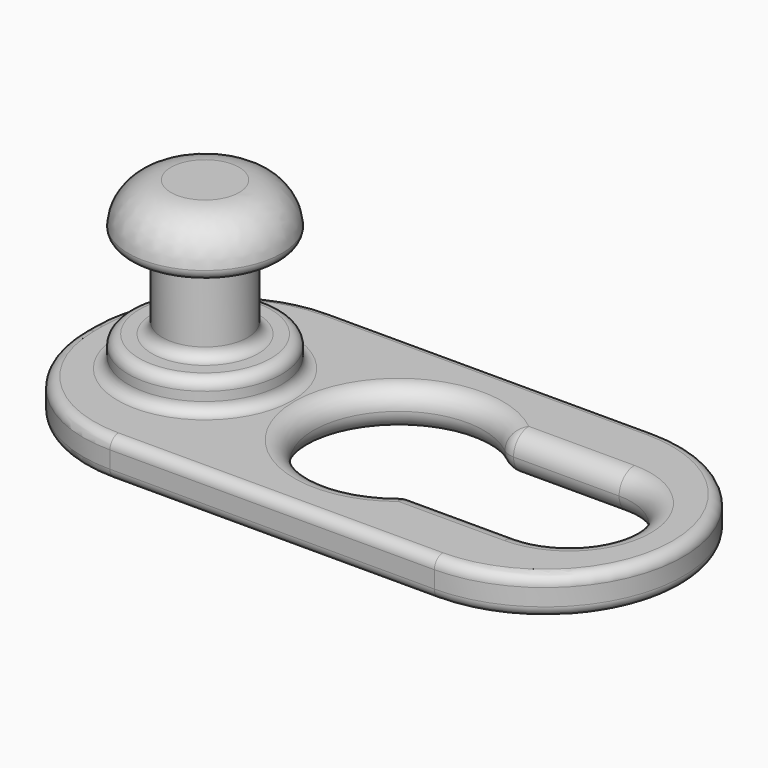
from build123d import *

# Parameters (mm, degrees)
F0_R     = 7.2
F1_DEPTH = 3.6
F2_R     = 1.79999
F3_R     = 7.2
F4_DEPTH = 6.45
F5_R     = 4
F6_DEPTH = 8
F8_R     = 1
F7_R     = 7.2
F7_R_2   = 4
F9_DEPTH = 4.75
F10_R    = 1
F12_R    = 1


# Not quite as in the source:
# - a fillet or chamfer that OpenCascade refuses, or shapes differently, is made with other operations: its cross-section is extruded or revolved along the edge and cut away or added
# - a fillet or chamfer is up to 0.001 mm smaller than in the source, because OpenCascade refuses the exact size


with BuildPart() as f1:
    # F0 (on Top) → F1 (new body)
    with BuildSketch(Plane.XY):
        with BuildLine():
            ThreePointArc((-17.2561568693, 13.0195750748), (-26.0949916342, 9.3584098397), (-29.7561568693, 0.5195750748))
            Line((-29.7561568693, 0.5195750748), (-29.7561568693, 0))
            Line((-29.7561568693, 0), (-29.7561568693, -0.4804249252))
            ThreePointArc((-29.7561568693, -0.4804249252), (-26.0949916342, -9.31925969), (-17.2561568693, -12.9804249252))
            Line((-17.2561568693, -12.9804249252), (13.2438431307, -12.9804249252))
            ThreePointArc((13.2438431307, -12.9804249252), (22.4362312861, -9.1728130806), (26.2438431307, 0.0195750748))
            ThreePointArc((26.2438431307, 0.0195750748), (22.4362312861, 9.2119632303), (13.2438431307, 13.0195750748))
            Line((13.2438431307, 13.0195750748), (-17.2561568693, 13.0195750748))
        make_face()
        with Locations((-18.7568739057, 0)):
            Circle(F0_R, mode=Mode.SUBTRACT)
        with BuildLine():
            ThreePointArc((4.956876454, -5.85), (-8.4999999419, 0), (4.956876454, 5.85))
            Line((4.956876454, 5.85), (5.4, 5.85))
            Line((5.4, 5.85), (15.5500000581, 5.85))
            ThreePointArc((15.5500000581, 5.85), (21.4000000581, 0), (15.5500000581, -5.85))
            Line((15.5500000581, -5.85), (5.4, -5.85))
            Line((5.4, -5.85), (4.956876454, -5.85))
        make_face(mode=Mode.SUBTRACT)
        with Locations((-18.7568739057, 0)):
            Circle(F0_R)
    extrude(amount=F1_DEPTH)

    # F2 (radius 1.8 in the source; OpenCascade refuses exactly that, so slightly less here)
    f2_edges = [f1.edges().sort_by_distance(p)[0] for p in [
        (4.956876, -5.85, 1.8),
        (4.956876, 5.85, 1.8),
        (-8.5, 0, 0),
        (-8.5, 0, 3.6),
        (15.55, 5.85, 1.8),
        (10.253438, 5.85, 0),
        (10.253438, 5.85, 3.6),
        (15.55, -5.85, 1.8),
        (21.4, 0, 0),
        (21.4, 0, 3.6),
        (10.253438, -5.85, 0),
        (10.253438, -5.85, 3.6),
    ]]
    fillet(f2_edges, radius=F2_R)

    # F3 (on Top) → F4 (join)
    with BuildSketch(Plane.XY):
        with Locations((-18.7010411173, 0)):
            Circle(F3_R)
    extrude(amount=F4_DEPTH)

    # F5 (on face) → F6 (join)
    with BuildSketch(Plane.XY.offset(6.45)):
        with Locations((-18.7010411173, 0)):
            Circle(F5_R)
    extrude(amount=F6_DEPTH)

    # F8
    f8_edges = [f1.edges().sort_by_distance(p)[0] for p in [
        (-25.901041, 0, 6.45),
        (-22.701041, 0, 6.45),
        (-25.901041, 0, 3.6),
        (-11.501041, 0, 5.025),
    ]]
    fillet(f8_edges, radius=F8_R)

    # F7 (on face) → F9 (join)
    with BuildSketch(Plane.XY.offset(14.45)):
        with Locations((-18.7010411173, 0)):
            Circle(F7_R)
        with Locations((-18.7010411173, 0)):
            Circle(F7_R_2, mode=Mode.SUBTRACT)
        with Locations((-18.7010411173, 0)):
            Circle(F7_R_2)
    extrude(amount=F9_DEPTH)

    # F10
    f10_edges = [f1.edges().sort_by_distance(p)[0] for p in [
        (-25.901041, 0, 14.45),
        (-22.701041, 0, 14.45),
        (-14.701041, 0, 10.95),
        (-22.701041, 0, 7.45),
    ]]
    fillet(f10_edges, radius=F10_R)

    # F11: fillet of radius 4 on 3 edges, made by hand

    # F11_s1 → F11_t2 (revolve, cut)
    with BuildSketch(Plane.XZ):
        with BuildLine():
            ThreePointArc((-11.5010411173, 15.45), (-12.7546081855, 18.1154759474), (-15.493220973, 19.2))
            Line((-15.493220973, 19.2), (-15.493220973, 19.28))
            Line((-15.493220973, 19.28), (-11.5010411173, 19.28))
            Line((-11.5010411173, 19.28), (-11.4210411173, 19.2))
            ThreePointArc((-11.4210411173, 19.2), (-11.4210411173, 17.325), (-11.4211975202, 15.455))
            Line((-11.4211975202, 15.455), (-11.5010411173, 15.45))
        make_face()
    revolve(axis=Axis((-18.7010411173, 0, 19.2), (0, 0, 1)), mode=Mode.SUBTRACT)

    # F12
    f12_edges = [f1.edges().sort_by_distance(p)[0] for p in [
        (-26.901041, 0, 3.6),
        (-26.094992, 9.35841, 3.6),
        (-2.006157, 13.019575, 3.6),
        (-29.756157, 0.019575, 3.6),
        (26.243843, 0.019575, 3.6),
        (-26.094992, -9.31926, 3.6),
        (-2.006157, -12.980425, 3.6),
        (-10.29999, 0, 3.6),
        (10.587575, -7.64999, 3.6),
        (10.587575, 7.64999, 3.6),
        (23.19999, 0, 3.6),
        (-29.756157, -0.480425, 1.8),
        (-17.256157, -12.980425, 1.8),
        (-26.094992, -9.31926, 0),
        (13.243843, -12.980425, 1.8),
        (-2.006157, -12.980425, 0),
        (13.243843, 13.019575, 1.8),
        (26.243843, 0.019575, 0),
        (-17.256157, 13.019575, 1.8),
        (-2.006157, 13.019575, 0),
        (-29.756157, 0.519575, 1.8),
        (-26.094992, 9.35841, 0),
        (-29.756157, 0.019575, 0),
    ]]
    fillet(f12_edges, radius=F12_R)


solid = f1.part
